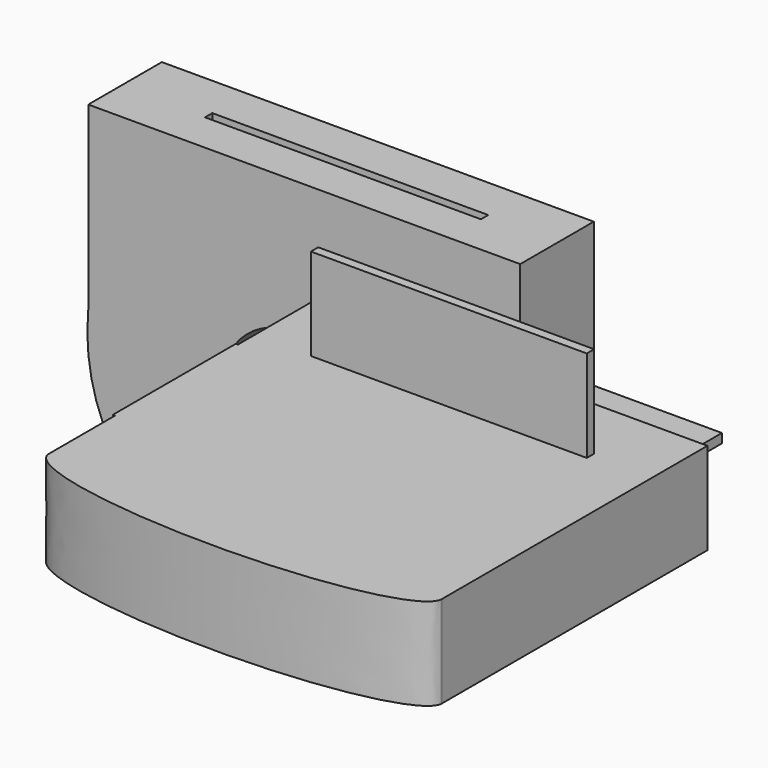
from build123d import *

# Parameters (mm, degrees)
F1_DEPTH = 25.4
F2_W     = 76.2
F2_H     = 2.54
F3_DEPTH = 25.4
F5_DEPTH = 25.4
F6_W     = 76.2
F6_H     = 2.54
F7_DEPTH = 25.4
F8_W     = 76.2
F8_H     = 2.54
F9_DEPTH = 25.4


with BuildPart() as f1:
    # F0 (on Front) → F1 (new body)
    with BuildSketch(Plane.XZ):
        with BuildLine():
            Line((62.2428618371, 51.8912672997), (-57.0498779416, 51.8912672997))
            Line((-57.0498779416, 51.8912672997), (-57.0498779416, 2.0486290034))
            add(Edge.make_bspline(
                [(-57.0498779416, 2.0486290034), (-62.8725917554, -57.5601651506), (-23.5538572735, -39.4474879084)],
                knots=[1.4290915848, 1.4290915848, 1.4290915848, 3.4471381657, 3.4471381657, 3.4471381657], degree=2, weights=[1, 0.5326875763, 1]))
            ThreePointArc((-23.5538572735, -39.4474879084), (-23.1311062984, -19.5726887681), (-19.6531451654, 0))
            ThreePointArc((-19.6531451654, 0), (0, 15.2158019665), (19.6531451654, 0))
            add(Edge.make_bspline(
                [(19.6531451654, 0), (20.6238584336, -3.4875863708), (22.5912929652, -10.5562008448), (24.2387527598, -21.9019388925), (24.1620099315, -33.4497913044), (24.11910519, -39.9058684707)],
                knots=[0, 0, 0, 0, 0.3004169931, 0.608882958, 1, 1, 1, 1], degree=3))
            add(Edge.make_bspline(
                [(47.476719356, -41.1129942258), (41.3063324166, -44.1182628579), (32.717853118, -42.0442846037), (24.11910519, -39.9058684707)],
                knots=[0.6578997811, 0.6578997811, 0.6578997811, 0.6578997811, 1, 1, 1, 1], degree=3))
            add(Edge.make_bspline(
                [(58.9949473098, -23.6284681863), (56.9882398729, -30.879237475), (53.3148096325, -38.2695696963), (47.476719356, -41.1129942258)],
                knots=[0.3342228414, 0.3342228414, 0.3342228414, 0.3342228414, 0.6578997811, 0.6578997811, 0.6578997811, 0.6578997811], degree=3))
            add(Edge.make_bspline(
                [(61.5792318695, -1.454491908), (61.36202452, -8.8032522142), (61.0670364179, -16.1414574779), (58.9949473098, -23.6284681863)],
                knots=[0, 0, 0, 0, 0.3342228414, 0.3342228414, 0.3342228414, 0.3342228414], degree=3))
            Line((61.5792318695, -1.454491908), (62.2428618371, 0))
            Line((62.2428618371, 0), (62.2428618371, 51.8912672997))
        make_face()
        with BuildLine():
            add(Edge.make_bspline(
                [(47.476719356, -41.1129942258), (57.185089489, -36.7539276341), (58.9949473098, -23.6284681863)],
                knots=[0.3330351725, 0.3330351725, 0.3330351725, 1.3936926102, 1.3936926102, 1.3936926102], degree=2, weights=[1, 0.8626408456, 1]))
            add(Edge.make_bspline(
                [(58.9949473098, -23.6284681863), (56.9882398729, -30.879237475), (53.3148096325, -38.2695696963), (47.476719356, -41.1129942258)],
                knots=[0.3342228414, 0.3342228414, 0.3342228414, 0.3342228414, 0.6578997811, 0.6578997811, 0.6578997811, 0.6578997811], degree=3))
        make_face()
    extrude(amount=F1_DEPTH)

    # F2 (on face) → F3 (cut)
    with BuildSketch(Plane.XY.offset(51.8912672997)):
        with Locations((4.4371271506, -13.0748547494)):
            Rectangle(F2_W, F2_H)
    extrude(amount=-F3_DEPTH, mode=Mode.SUBTRACT)


with BuildPart() as f5:
    # F4 (on Top) → F5 (new body)
    with BuildSketch(Plane.XY):
        with BuildLine():
            Line((6.4240375055, -95.4406112065), (6.4240375055, -118.3726499874))
            add(Edge.make_bspline(
                [(6.4240375055, -118.3726499874), (6.4240375055, -118.5430909379), (6.4487490888, -118.7134542936)],
                knots=[3.1415926536, 3.1415926536, 3.1415926536, 3.1717686083, 3.1717686083, 3.1717686083], degree=2, weights=[1, 0.9998861786, 1]))
            add(Edge.make_bspline(
                [(6.4487490888, -118.7134542936), (8.0377690426, -129.6682672247), (60.7042431856, -129.6682672247), (113.3707173286, -129.6682672247), (114.9597372824, -118.7134542936)],
                knots=[3.1717686083, 3.1717686083, 3.1717686083, 4.7123889804, 4.7123889804, 6.2530093525, 6.2530093525, 6.2530093525], degree=2, weights=[1, 0.7176947036, 1, 0.7176947036, 1]))
            add(Edge.make_bspline(
                [(114.9597372824, -118.7134542936), (114.9844488657, -118.5430909379), (114.9844488657, -118.3726499874)],
                knots=[6.2530093525, 6.2530093525, 6.2530093525, 6.2831853072, 6.2831853072, 6.2831853072], degree=2, weights=[1, 0.9998861786, 1]))
            Line((114.9844488657, -118.3726499874), (114.9844488657, -95.4406112065))
            Line((114.9844488657, -95.4406112065), (114.9844488657, -53.0177001276))
            Line((114.9844488657, -53.0177001276), (114.9844488657, -26.7026225953))
            Line((114.9844488657, -26.7026225953), (6.38557814, -26.7026225953))
            Line((6.38557814, -26.7026225953), (6.38557814, -53.0177001276))
            Line((6.38557814, -53.0177001276), (5.8152723915, -53.0177001276))
            Line((5.8152723915, -53.0177001276), (5.8152723915, -95.4406112065))
            Line((5.8152723915, -95.4406112065), (6.4240375055, -95.4406112065))
        make_face()
    extrude(amount=F5_DEPTH)

    # F6 (on face) → F7 (join)
    with BuildSketch(Plane.XY.offset(25.4)):
        with Locations((60.1108064875, -46.1128767049)):
            Rectangle(F6_W, F6_H)
    extrude(amount=F7_DEPTH)

    # F8 (on face) → F9 (join)
    with BuildSketch(Plane(origin=(0, -26.7026225953, 0), x_dir=(-1, 0, 0), z_dir=(0, 1, 0))):
        with Locations((-60.5735373735, 11.6173765776)):
            Rectangle(F8_W, F8_H)
    extrude(amount=F9_DEPTH)


solid = Compound([f1.part, f5.part])
